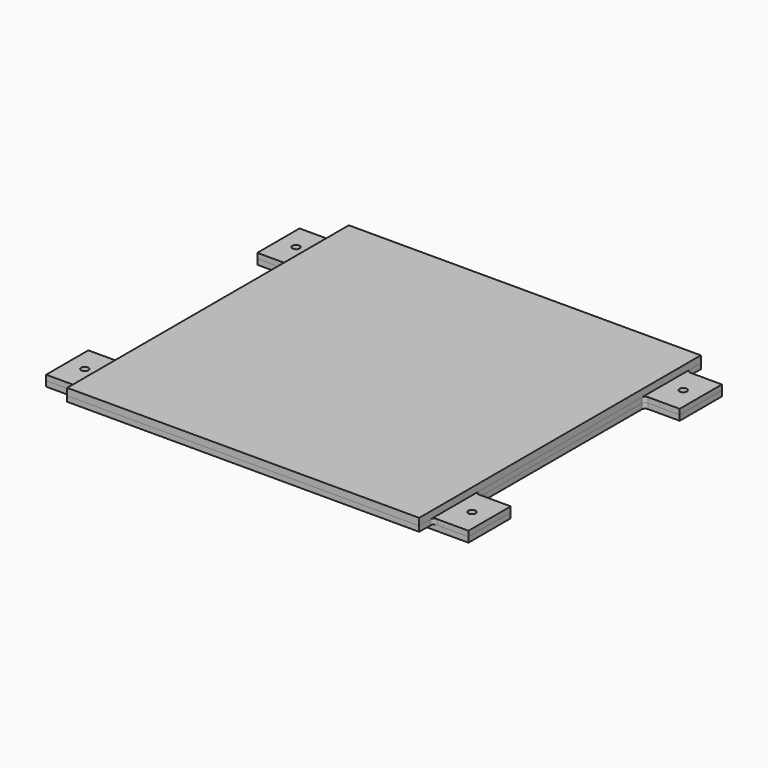
from build123d import *

# Parameters (mm, degrees)
F0_R     = 2.1
F0_R_2   = 2.6
F0_R_3   = 65
F1_DEPTH = 3
F2_R     = 2.1
F2_R_2   = 2.6
F2_R_3   = 65
F3_DEPTH = 3
F5_DEPTH = 4


with BuildPart() as f1:
    # F0 (on Top) → F1 (new body)
    with BuildSketch(Plane.XY):
        with BuildLine():
            Line((-120, -60), (-120, -90))
            Line((-120, -90), (-102, -90))
            Line((-102, -90), (-22.360679775, -90))
            ThreePointArc((-22.360679775, -90), (0, -80), (22.360679775, -90))
            Line((22.360679775, -90), (102, -90))
            Line((102, -90), (120, -90))
            Line((120, -90), (120, -60))
            Line((120, -60), (102, -60))
            ThreePointArc((102, -60), (100.5857864376, -59.4142135624), (100, -58))
            Line((100, -58), (100, 58))
            ThreePointArc((100, 58), (100.5857864376, 59.4142135624), (102, 60))
            Line((102, 60), (120, 60))
            Line((120, 60), (120, 90))
            Line((120, 90), (102, 90))
            Line((102, 90), (22.360679775, 90))
            ThreePointArc((22.360679775, 90), (0, 80), (-22.360679775, 90))
            Line((-22.360679775, 90), (-102, 90))
            Line((-102, 90), (-120, 90))
            Line((-120, 90), (-120, 60))
            Line((-120, 60), (-102, 60))
            ThreePointArc((-102, 60), (-100.5857864376, 59.4142135624), (-100, 58))
            Line((-100, 58), (-100, -58))
            ThreePointArc((-100, -58), (-100.5857864376, -59.4142135624), (-102, -60))
            Line((-102, -60), (-120, -60))
        make_face()
        with Locations((-110, -75)):
            Circle(F0_R, mode=Mode.SUBTRACT)
        with Locations((-79, -75)):
            Circle(F0_R_2, mode=Mode.SUBTRACT)
        with Locations((79, -75)):
            Circle(F0_R_2, mode=Mode.SUBTRACT)
        with Locations((110, -75)):
            Circle(F0_R, mode=Mode.SUBTRACT)
        with Locations((-110, 75)):
            Circle(F0_R, mode=Mode.SUBTRACT)
        with Locations((-79, 75)):
            Circle(F0_R_2, mode=Mode.SUBTRACT)
        Circle(F0_R_3, mode=Mode.SUBTRACT)
        with Locations((79, 75)):
            Circle(F0_R_2, mode=Mode.SUBTRACT)
        with Locations((110, 75)):
            Circle(F0_R, mode=Mode.SUBTRACT)
    extrude(amount=F1_DEPTH)


with BuildPart() as f3:
    # F2 (on face) → F3 (new body)
    with BuildSketch(Plane.XY.offset(3)):
        with BuildLine():
            Line((-22.360679775, 90), (-102, 90))
            Line((-102, 90), (-120, 90))
            Line((-120, 90), (-120, 60))
            Line((-120, 60), (-102, 60))
            ThreePointArc((-102, 60), (-100.5857864376, 59.4142135624), (-100, 58))
            Line((-100, 58), (-100, -58))
            ThreePointArc((-100, -58), (-100.5857864376, -59.4142135624), (-102, -60))
            Line((-102, -60), (-120, -60))
            Line((-120, -60), (-120, -90))
            Line((-120, -90), (-102, -90))
            Line((-102, -90), (-22.360679775, -90))
            ThreePointArc((-22.360679775, -90), (0, -80), (22.360679775, -90))
            Line((22.360679775, -90), (102, -90))
            Line((102, -90), (120, -90))
            Line((120, -90), (120, -60))
            Line((120, -60), (102, -60))
            ThreePointArc((102, -60), (100.5857864376, -59.4142135624), (100, -58))
            Line((100, -58), (100, 58))
            ThreePointArc((100, 58), (100.5857864376, 59.4142135624), (102, 60))
            Line((102, 60), (120, 60))
            Line((120, 60), (120, 90))
            Line((120, 90), (102, 90))
            Line((102, 90), (22.360679775, 90))
            ThreePointArc((22.360679775, 90), (0, 80), (-22.360679775, 90))
        make_face()
        with Locations((-110, -75)):
            Circle(F2_R, mode=Mode.SUBTRACT)
        with Locations((-79, -75)):
            Circle(F2_R_2, mode=Mode.SUBTRACT)
        with Locations((79, -75)):
            Circle(F2_R_2, mode=Mode.SUBTRACT)
        with Locations((110, -75)):
            Circle(F2_R, mode=Mode.SUBTRACT)
        with Locations((-110, 75)):
            Circle(F2_R, mode=Mode.SUBTRACT)
        with Locations((-79, 75)):
            Circle(F2_R_2, mode=Mode.SUBTRACT)
        Circle(F2_R_3, mode=Mode.SUBTRACT)
        with Locations((79, 75)):
            Circle(F2_R_2, mode=Mode.SUBTRACT)
        with Locations((110, 75)):
            Circle(F2_R, mode=Mode.SUBTRACT)
        with BuildLine():
            Line((100, 100), (-100, 100))
            Line((-100, 100), (-100, 92))
            ThreePointArc((-100, 92), (-100.5857864376, 90.5857864376), (-102, 90))
            Line((-102, 90), (-22.360679775, 90))
            ThreePointArc((-22.360679775, 90), (0, 80), (22.360679775, 90))
            Line((22.360679775, 90), (102, 90))
            ThreePointArc((102, 90), (100.5857864376, 90.5857864376), (100, 92))
            Line((100, 92), (100, 100))
        make_face()
        with Locations((-79, 75)):
            Circle(F2_R_2)
        Circle(F2_R_3)
        with Locations((79, 75)):
            Circle(F2_R_2)
        with Locations((79, -75)):
            Circle(F2_R_2)
        with BuildLine():
            Line((-22.360679775, -90), (-102, -90))
            ThreePointArc((-102, -90), (-100.5857864376, -90.5857864376), (-100, -92))
            Line((-100, -92), (-100, -100))
            Line((-100, -100), (100, -100))
            Line((100, -100), (100, -92))
            ThreePointArc((100, -92), (100.5857864376, -90.5857864376), (102, -90))
            Line((102, -90), (22.360679775, -90))
            ThreePointArc((22.360679775, -90), (0, -80), (-22.360679775, -90))
        make_face()
        with Locations((-79, -75)):
            Circle(F2_R_2)
    extrude(amount=F3_DEPTH)


with BuildPart() as f5:
    # F4 (on face) → F5 (new body)
    with BuildSketch(Plane.XY.offset(6)):
        Polygon((100, 100), (-100, 100), (-100, 92), (-100, 58), (-100, -58), (-100, -92), (-100, -100), (100, -100), (100, -92), (100, -58), (100, 58), (100, 92), align=None)
    extrude(amount=F5_DEPTH)


solid = Compound([f1.part, f3.part, f5.part])
